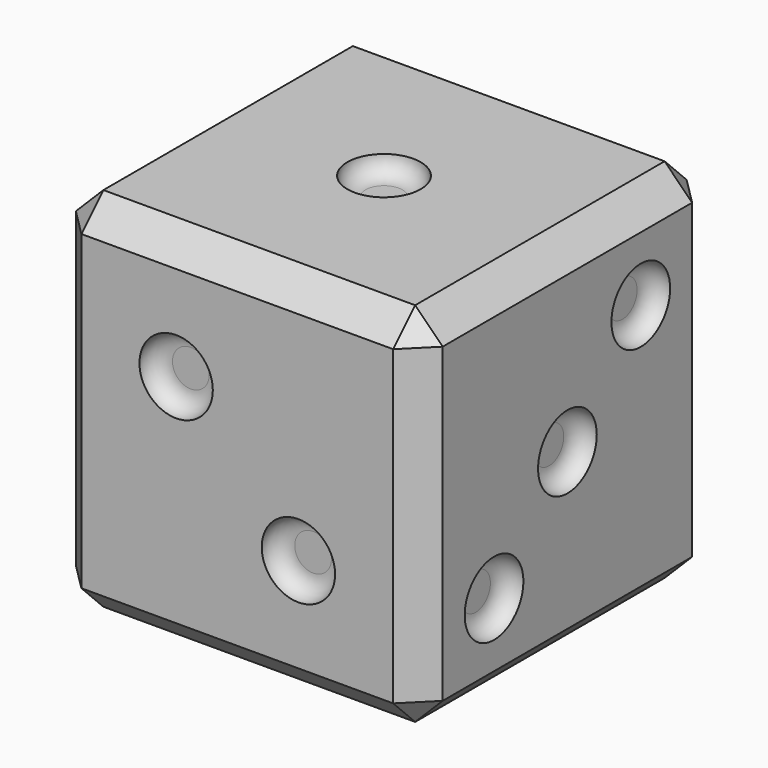
from build123d import *

# Parameters (mm, degrees)
F0_W      = 20
F0_H      = 20
F1_DEPTH  = 20
F5_R      = 2
F8_DEPTH  = 1
F2_R      = 2
F9_DEPTH  = 1
F3_R      = 2
F10_DEPTH = 1
F7_R      = 2
F11_DEPTH = 1
F4_R      = 2
F12_DEPTH = 1
F6_R      = 2
F13_DEPTH = 1
F14_SIZE  = 1.5
F15_R     = 0.99999


# Not quite as in the source:
# - a fillet or chamfer is up to 0.001 mm smaller than in the source, because OpenCascade refuses the exact size


with BuildPart() as f1:
    # F0 (on Top) → F1 (new body)
    with BuildSketch(Plane.XY):
        with Locations((10, 10)):
            Rectangle(F0_W, F0_H)
    extrude(amount=F1_DEPTH)

    # F5 (on face) → F8 (cut)
    with BuildSketch(Plane(origin=(0, 20, 0), x_dir=(-1, 0, 0), z_dir=(0, 1, 0))):
        with Locations((-16, 16)):
            Circle(F5_R)
        with Locations((-4, 16)):
            Circle(F5_R)
        with Locations((-10, 10)):
            Circle(F5_R)
        with Locations((-4, 4)):
            Circle(F5_R)
        with Locations((-16, 4)):
            Circle(F5_R)
    extrude(amount=-F8_DEPTH, mode=Mode.SUBTRACT)

    # F2 (on face) → F9 (cut)
    with BuildSketch(Plane.XY.offset(20)):
        with Locations((10, 10)):
            Circle(F2_R)
    extrude(amount=-F9_DEPTH, mode=Mode.SUBTRACT)

    # F3 (on face) → F10 (cut)
    with BuildSketch(Plane(origin=(0, 0, 0), x_dir=(1, 0, 0), z_dir=(0, 0, -1))):
        with Locations((16, -16)):
            Circle(F3_R)
        with Locations((16, -10)):
            Circle(F3_R)
        with Locations((16, -4)):
            Circle(F3_R)
        with Locations((4, -4)):
            Circle(F3_R)
        with Locations((4, -10)):
            Circle(F3_R)
        with Locations((4, -16)):
            Circle(F3_R)
    extrude(amount=-F10_DEPTH, mode=Mode.SUBTRACT)

    # F7 (on face) → F11 (cut)
    with BuildSketch(Plane(origin=(0, 0, 0), x_dir=(0, -1, 0), z_dir=(-1, 0, 0))):
        with Locations((-16, 4)):
            Circle(F7_R)
        with Locations((-16, 16)):
            Circle(F7_R)
        with Locations((-4, 16)):
            Circle(F7_R)
        with Locations((-4, 4)):
            Circle(F7_R)
    extrude(amount=-F11_DEPTH, mode=Mode.SUBTRACT)

    # F4 (on face) → F12 (cut)
    with BuildSketch(Plane.XZ):
        with Locations((13.3333333333, 6.6666666667)):
            Circle(F4_R)
        with Locations((6.6666666667, 13.3333333333)):
            Circle(F4_R)
    extrude(amount=-F12_DEPTH, mode=Mode.SUBTRACT)

    # F6 (on face) → F13 (cut)
    with BuildSketch(Plane.YZ.offset(20)):
        with Locations((15, 15)):
            Circle(F6_R)
        with Locations((10, 10)):
            Circle(F6_R)
        with Locations((5, 5)):
            Circle(F6_R)
    extrude(amount=-F13_DEPTH, mode=Mode.SUBTRACT)

    # F14
    f14_edges = [f1.edges().sort_by_distance(p)[0] for p in [
        (20, 10, 20),
        (20, 0, 10),
        (20, 20, 10),
        (20, 10, 0),
        (10, 0, 0),
        (10, 20, 0),
        (0, 10, 0),
        (0, 0, 10),
        (10, 0, 20),
        (10, 20, 20),
        (0, 20, 10),
        (0, 10, 20),
    ]]
    chamfer(f14_edges, length=F14_SIZE)

    # F15 (radius 1 in the source; OpenCascade refuses exactly that, so slightly less here)
    f15_edges = [f1.edges().sort_by_distance(p)[0] for p in [
        (6, 19, 16),
        (12, 19, 10),
        (18, 19, 16),
        (18, 19, 4),
        (6, 19, 4),
        (19, 13, 15),
        (19, 8, 10),
        (19, 3, 5),
        (8, 10, 19),
        (1, 18, 16),
        (1, 18, 4),
        (1, 6, 4),
        (1, 6, 16),
        (4.666667, 1, 13.333333),
        (11.333333, 1, 6.666667),
        (2, 4, 1),
        (2, 10, 1),
        (2, 16, 1),
        (14, 16, 1),
        (14, 10, 1),
        (14, 4, 1),
    ]]
    fillet(f15_edges, radius=F15_R)


solid = f1.part
